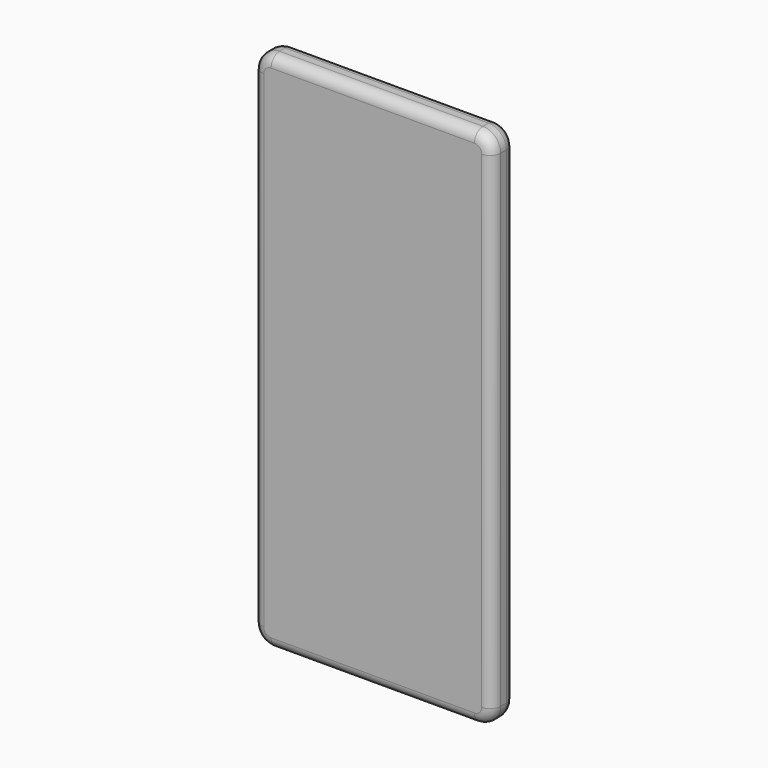
from build123d import *

# Parameters (mm, degrees)
F0_W         = 68.1
F0_H         = 148.9
F1_DEPTH     = 8
F2_R         = 3
F3_R         = 3
F4_T1_DEPTH  = 8
F4_T4_ANGLE  = 90
F4_T6_ANGLE  = 90
F5_T1_DEPTH  = 8
F5_T4_ANGLE  = 90
F5_T6_ANGLE  = 90
F5_T8_ANGLE  = 90
F5_T10_ANGLE = 90
F5_T12_ANGLE = 90
F5_T14_ANGLE = 90


# Not quite as in the source:
# - a fillet or chamfer that OpenCascade refuses, or shapes differently, is made with other operations: its cross-section is extruded or revolved along the edge and cut away or added


with BuildPart() as f1:
    # F0 (on Front) → F1 (new body)
    with BuildSketch(Plane.XZ):
        with Locations((7.5711421669, 34.216450589)):
            Rectangle(F0_W, F0_H)
    extrude(amount=F1_DEPTH)

    # F2
    f2_edges = [f1.edges().sort_by_distance(p)[0] for p in [
        (41.621142, -8, 34.216451),
        (7.571142, -8, 108.666451),
        (-26.478858, -8, 34.216451),
        (7.571142, -8, -40.233549),
    ]]
    fillet(f2_edges, radius=F2_R)

    # F3
    f3_edges = [f1.edges().sort_by_distance(p)[0] for p in [
        (41.621142, 0, 34.216451),
        (7.571142, 0, 108.666451),
        (-26.478858, 0, 34.216451),
        (7.571142, 0, -40.233549),
    ]]
    fillet(f3_edges, radius=F3_R)

    # F4: fillet of radius 5.08 on 1 edges, made by hand

    # F4_s2 → F4_t1 (cut)
    with BuildSketch(Plane.XZ):
        with BuildLine():
            ThreePointArc((41.6211421669, -35.153549411), (40.1332446153, -38.7456518594), (36.5411421669, -40.233549411))
            Line((36.5411421669, -40.233549411), (41.6211421669, -40.233549411))
            Line((41.6211421669, -40.233549411), (41.6211421669, -35.153549411))
        make_face()
    extrude(amount=F4_T1_DEPTH, mode=Mode.SUBTRACT)

    # F4_s3 → F4_t4 (revolve, cut)
    with BuildSketch(Plane.YZ.offset(36.5411421669)):
        with BuildLine():
            ThreePointArc((-8, -37.233549411), (-7.1213203436, -39.3548697546), (-5, -40.233549411))
            Line((-5, -40.233549411), (-8, -40.233549411))
            Line((-8, -40.233549411), (-8, -37.233549411))
        make_face()
    revolve(axis=Axis((36.5411421669, -8, -35.153549411), (0, -1, 0)), revolution_arc=F4_T4_ANGLE, mode=Mode.SUBTRACT)

    # F4_s5 → F4_t6 (revolve, cut)
    with BuildSketch(Plane.XY.offset(-35.153549411)):
        with BuildLine():
            ThreePointArc((38.6211421669, 0), (40.7424625104, -0.8786796564), (41.6211421669, -3))
            Line((41.6211421669, -3), (41.6211421669, 0))
            Line((41.6211421669, 0), (38.6211421669, 0))
        make_face()
    revolve(axis=Axis((36.5411421669, 0, -35.153549411), (0, 1, 0)), revolution_arc=F4_T6_ANGLE, mode=Mode.SUBTRACT)

    # F5: fillet of radius 5.08 on 3 edges, made by hand

    # F5_s2 → F5_t1 (cut)
    with BuildSketch(Plane.XZ):
        with BuildLine():
            ThreePointArc((-26.4788578331, -35.153549411), (-24.9909602816, -38.7456518594), (-21.3988578331, -40.233549411))
            Line((-21.3988578331, -40.233549411), (-26.4788578331, -40.233549411))
            Line((-26.4788578331, -40.233549411), (-26.4788578331, -35.153549411))
        make_face()
        with BuildLine():
            ThreePointArc((-21.3988578331, 108.666450589), (-24.9909602816, 107.1785530374), (-26.4788578331, 103.586450589))
            Line((-26.4788578331, 103.586450589), (-26.4788578331, 108.666450589))
            Line((-26.4788578331, 108.666450589), (-21.3988578331, 108.666450589))
        make_face()
        with BuildLine():
            ThreePointArc((41.6211421669, 103.586450589), (40.1332446153, 107.1785530374), (36.5411421669, 108.666450589))
            Line((36.5411421669, 108.666450589), (41.6211421669, 108.666450589))
            Line((41.6211421669, 108.666450589), (41.6211421669, 103.586450589))
        make_face()
    extrude(amount=F5_T1_DEPTH, mode=Mode.SUBTRACT)

    # F5_s3 → F5_t4 (revolve, cut)
    with BuildSketch(Plane.YZ.offset(36.5411421669)):
        with BuildLine():
            ThreePointArc((0, 105.666450589), (-0.8786796564, 107.7877709326), (-3, 108.666450589))
            Line((-3, 108.666450589), (0, 108.666450589))
            Line((0, 108.666450589), (0, 105.666450589))
        make_face()
    revolve(axis=Axis((36.5411421669, 0, 103.586450589), (0, 1, 0)), revolution_arc=F5_T4_ANGLE, mode=Mode.SUBTRACT)

    # F5_s5 → F5_t6 (revolve, cut)
    with BuildSketch(Plane.XY.offset(103.586450589)):
        with BuildLine():
            ThreePointArc((38.6211421669, -8), (40.7424625104, -7.1213203436), (41.6211421669, -5))
            Line((41.6211421669, -5), (41.6211421669, -8))
            Line((41.6211421669, -8), (38.6211421669, -8))
        make_face()
    revolve(axis=Axis((36.5411421669, -8, 103.586450589), (0, -1, 0)), revolution_arc=F5_T6_ANGLE, mode=Mode.SUBTRACT)

    # F5_s7 → F5_t8 (revolve, cut)
    with BuildSketch(Plane.XY.offset(103.586450589)):
        with BuildLine():
            ThreePointArc((-23.4788578331, 0), (-25.6001781767, -0.8786796564), (-26.4788578331, -3))
            Line((-26.4788578331, -3), (-26.4788578331, 0))
            Line((-26.4788578331, 0), (-23.4788578331, 0))
        make_face()
    revolve(axis=Axis((-21.3988578331, 0, 103.586450589), (0, 1, 0)), revolution_arc=F5_T8_ANGLE, mode=Mode.SUBTRACT)

    # F5_s9 → F5_t10 (revolve, cut)
    with BuildSketch(Plane.YZ.offset(-21.3988578331)):
        with BuildLine():
            ThreePointArc((-8, 105.666450589), (-7.1213203436, 107.7877709326), (-5, 108.666450589))
            Line((-5, 108.666450589), (-8, 108.666450589))
            Line((-8, 108.666450589), (-8, 105.666450589))
        make_face()
    revolve(axis=Axis((-21.3988578331, -8, 103.586450589), (0, -1, 0)), revolution_arc=F5_T10_ANGLE, mode=Mode.SUBTRACT)

    # F5_s11 → F5_t12 (revolve, cut)
    with BuildSketch(Plane.YZ.offset(-21.3988578331)):
        with BuildLine():
            ThreePointArc((0, -37.233549411), (-0.8786796564, -39.3548697546), (-3, -40.233549411))
            Line((-3, -40.233549411), (0, -40.233549411))
            Line((0, -40.233549411), (0, -37.233549411))
        make_face()
    revolve(axis=Axis((-21.3988578331, 0, -35.153549411), (0, 1, 0)), revolution_arc=F5_T12_ANGLE, mode=Mode.SUBTRACT)

    # F5_s13 → F5_t14 (revolve, cut)
    with BuildSketch(Plane.XY.offset(-35.153549411)):
        with BuildLine():
            ThreePointArc((-23.4788578331, -8), (-25.6001781767, -7.1213203436), (-26.4788578331, -5))
            Line((-26.4788578331, -5), (-26.4788578331, -8))
            Line((-26.4788578331, -8), (-23.4788578331, -8))
        make_face()
    revolve(axis=Axis((-21.3988578331, -8, -35.153549411), (0, -1, 0)), revolution_arc=F5_T14_ANGLE, mode=Mode.SUBTRACT)


solid = f1.part
